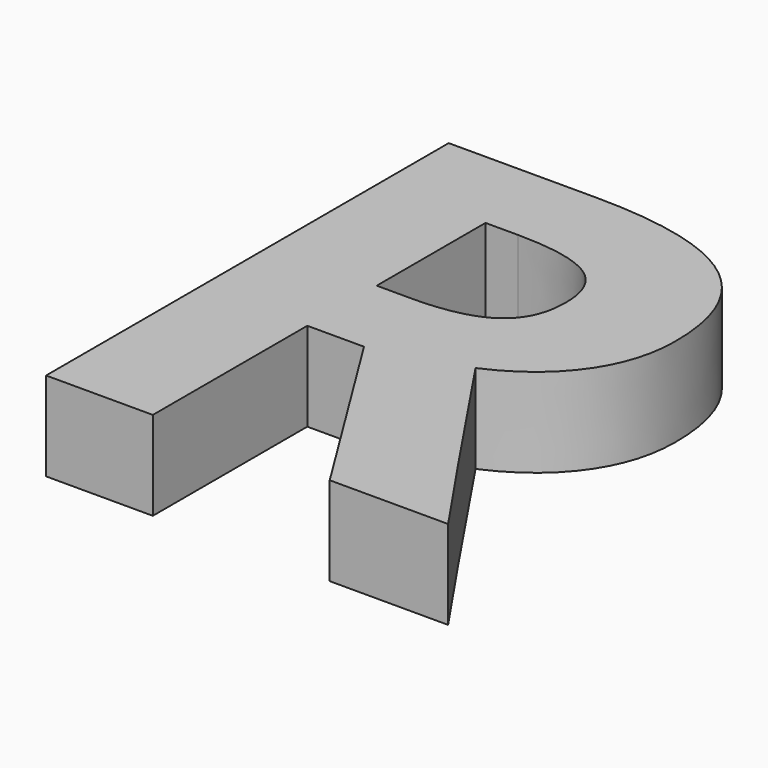
from build123d import *

# Parameters (mm, degrees)
F0_TEXT_SIZE = 79.3542454226
F1_DEPTH     = 10


# Not quite as in the source:
# - Text() gives the source's letters only with a copy of the font that has no kerning and outlines rounded to 1/6400 em; it was checked with that copy


with BuildPart() as f1:
    # F0 (on Top) → F1 (new body)
    with BuildSketch(Plane.XY):
        with Locations((0, 0)):
            Text('R', F0_TEXT_SIZE, font='Open Sans', font_style=FontStyle.BOLD, text_align=(TextAlign.LEFT, TextAlign.BOTTOM))
    extrude(amount=F1_DEPTH)


solid = f1.part
